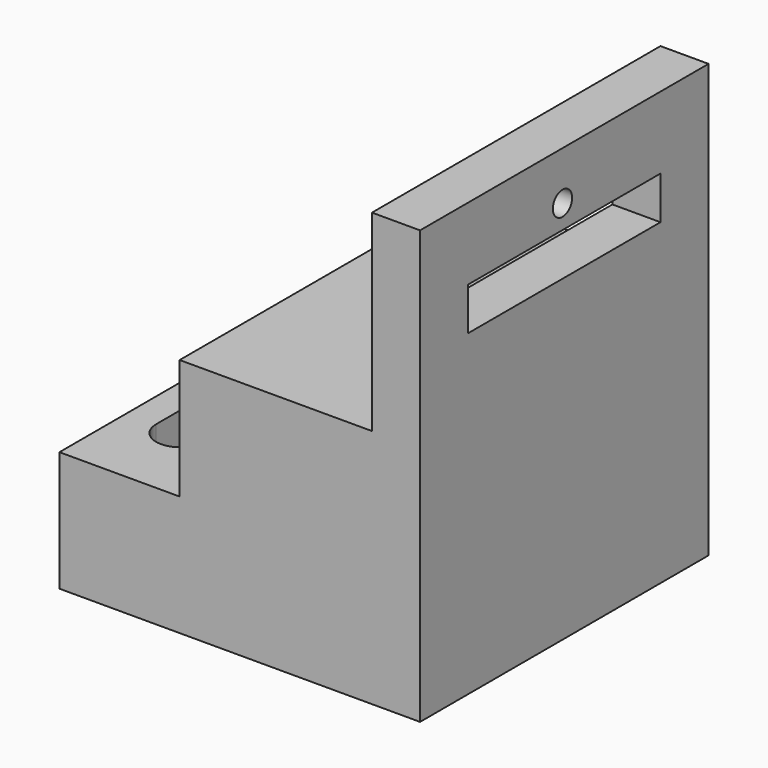
from build123d import *

# Parameters (mm, degrees)
F1_DEPTH = 150
F2_R     = 5
F3_DEPTH = 20.001
F4_W     = 100
F4_H     = 17.8262033769
F5_DEPTH = 20.001
F7_DEPTH = 25


with BuildPart() as f1:
    # F0 (on Front) → F1 (new body)
    with BuildSketch(Plane.XZ):
        Polygon((75, -90), (75, 90), (55, 90), (55, 10), (-25, 10), (-25, -40), (-75, -40), (-75, -90), align=None)
    extrude(amount=F1_DEPTH)

    # F2 (on face) → F3 (cut, through all)
    with BuildSketch(Plane(origin=(55, 0, 0), x_dir=(0, -1, 0), z_dir=(-1, 0, 0))):
        with Locations((75.9465023875, 69.8286518455)):
            Circle(F2_R)
    extrude(amount=-F3_DEPTH, mode=Mode.SUBTRACT)

    # F4 (on face) → F5 (cut, through all)
    with BuildSketch(Plane(origin=(55, 0, 0), x_dir=(0, -1, 0), z_dir=(-1, 0, 0))):
        with Locations((75, 51.0868983116)):
            Rectangle(F4_W, F4_H)
    extrude(amount=-F5_DEPTH, mode=Mode.SUBTRACT)

    # F6 (on face) → F7 (cut)
    with BuildSketch(Plane.XY.offset(-40)):
        with BuildLine():
            ThreePointArc((-42.7634136379, -115), (-52.7634136379, -105), (-62.7634136379, -115))
            Line((-62.7634136379, -115), (-42.7634136379, -115))
        make_face()
        with BuildLine():
            Line((-62.7634136379, -35), (-62.7634136379, -115))
            ThreePointArc((-62.7634136379, -115), (-52.7634136379, -105), (-42.7634136379, -115))
            Line((-42.7634136379, -115), (-42.7634136379, -35))
            ThreePointArc((-42.7634136379, -35), (-52.7634136379, -45), (-62.7634136379, -35))
        make_face()
        with BuildLine():
            Line((-42.7634136379, -115), (-62.7634136379, -115))
            ThreePointArc((-62.7634136379, -115), (-52.7634136379, -125), (-42.7634136379, -115))
        make_face()
        with BuildLine():
            ThreePointArc((-42.7634136379, -35), (-52.7634136379, -25), (-62.7634136379, -35))
            Line((-62.7634136379, -35), (-42.7634136379, -35))
        make_face()
        with BuildLine():
            Line((-42.7634136379, -35), (-62.7634136379, -35))
            ThreePointArc((-62.7634136379, -35), (-52.7634136379, -45), (-42.7634136379, -35))
        make_face()
    extrude(amount=-F7_DEPTH, mode=Mode.SUBTRACT)


solid = f1.part
